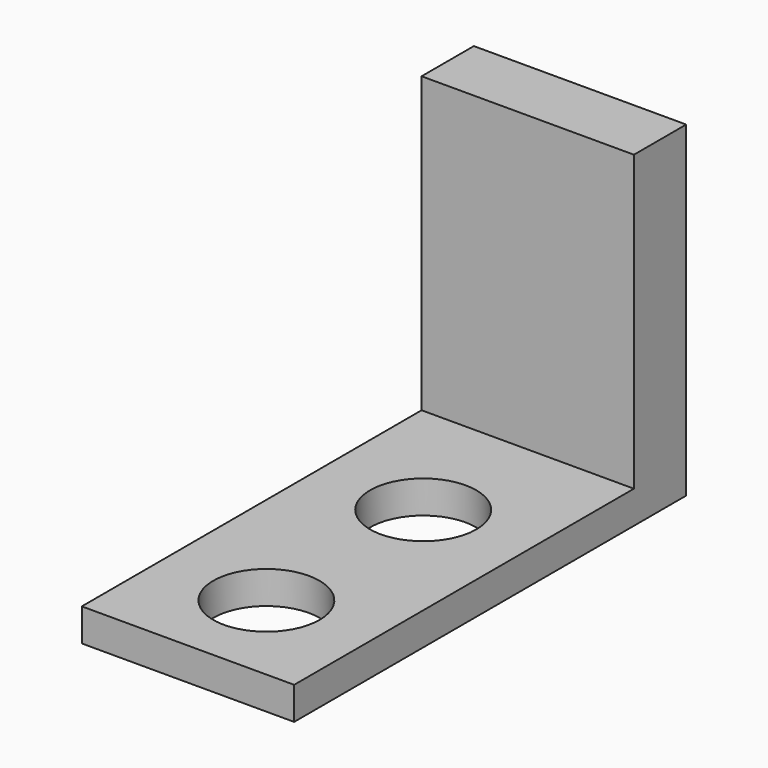
from build123d import *

# Parameters (mm, degrees)
F0_W     = 82.55
F0_H     = 12.7
F1_DEPTH = 190.5
F2_R     = 20.6375
F4_DEPTH = 25.4
F5_W     = 82.55
F5_H     = 25.4
F7_DEPTH = 114.3


with BuildPart() as f1:
    # F0 (on Front) → F1 (new body)
    with BuildSketch(Plane.XZ):
        with Locations((41.275, 6.35)):
            Rectangle(F0_W, F0_H)
    extrude(amount=F1_DEPTH)

    # F2 (on face) → F4 (cut)
    with BuildSketch(Plane(origin=(0, 0, 0), x_dir=(1, 0, 0), z_dir=(0, 0, -1))):
        with Locations((41.275, 76.2)):
            Circle(F2_R)
        with Locations((41.275, 152.4)):
            Circle(F2_R)
    extrude(amount=-F4_DEPTH, mode=Mode.SUBTRACT)

    # F5 (on face) → F7 (join)
    with BuildSketch(Plane.XY.offset(12.7)):
        with Locations((41.275, -12.7)):
            Rectangle(F5_W, F5_H)
    extrude(amount=F7_DEPTH)


solid = f1.part
